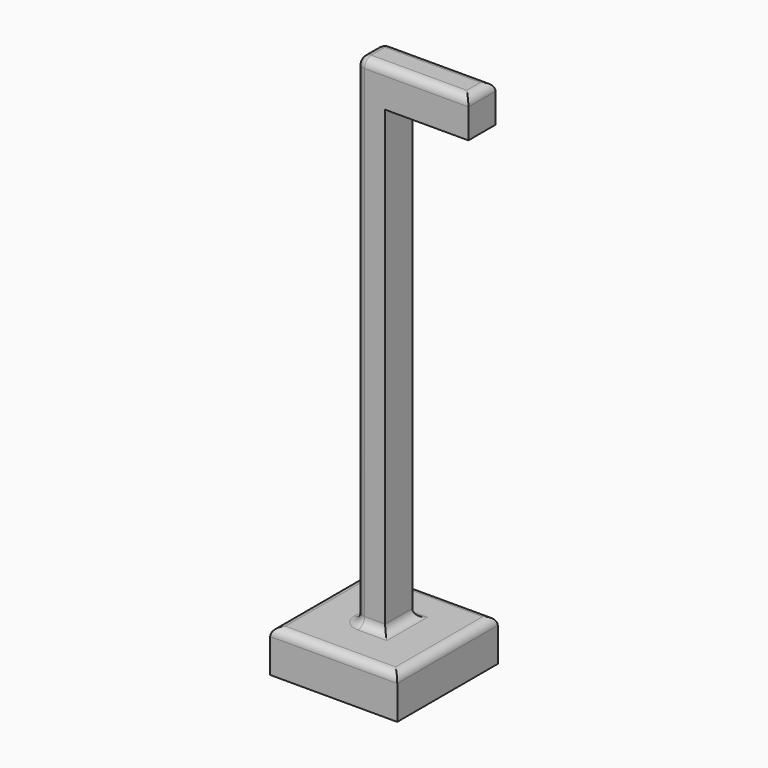
from build123d import *

# Parameters (mm, degrees)
F0_W        = 76.344192028
F0_H        = 75.5144134164
F1_DEPTH    = 25.4
F2_W        = 17.4319148064
F2_H        = 20.3372240067
F3_DEPTH    = 300
F4_W        = 20.3372240067
F4_H        = 22.7871290684
F5_DEPTH    = 50
F6_F1_R     = 5.08
F6_F2_R     = 5.08
F7_T        = 2.54
F7_T3_DEPTH = 10.16
F7_T5_DEPTH = 25.4172240067
F7_T7_DEPTH = 10.16
F8_R        = 5.08


# Not quite as in the source:
# - a shell that OpenCascade refuses in one call is made with other operations: the cavity is built on its own and cut out


with BuildPart() as f1:
    # F0 (on Top) → F1 (new body)
    with BuildSketch(Plane.XY):
        with Locations((38.172096014, 37.7572067082)):
            Rectangle(F0_W, F0_H)
    extrude(amount=F1_DEPTH)

    # F2 (on face) → F3 (join)
    with BuildSketch(Plane.XY.offset(25.4)):
        with Locations((37.6336574554, 38.5992005467)):
            Rectangle(F2_W, F2_H)
    extrude(amount=F3_DEPTH)

    # F4 (on face) → F5 (join)
    with BuildSketch(Plane.YZ.offset(46.3496148586)):
        with Locations((38.5992005467, 314.0064354658)):
            Rectangle(F4_W, F4_H)
    extrude(amount=F5_DEPTH)

    # F6: fillet of radius 5.08 on 7 edges, made by hand

    # F6_f1
    f6_f1_edges = [f1.edges().sort_by_distance(p)[0] for p in [
        (28.9177000523, 48.7678125501, 175.4),
        (28.9177000523, 28.4305885434, 175.4),
        (28.9177000523, 38.5992005467, 325.4),
        (62.6336574554, 48.7678125501, 325.4),
        (62.6336574554, 28.4305885434, 325.4),
        (96.3496148586, 38.5992005467, 325.4),
    ]]
    fillet(f6_f1_edges, radius=F6_F1_R)

    # F6_f2
    f6_f2_edges = [f1.edges().sort_by_distance(p)[0] for p in [
        (28.9177000523, 38.5992005467, 25.4),
        (30.4055976038, 47.2799149985, 25.4),
        (30.4055976038, 29.918486095, 25.4),
    ]]
    fillet(f6_f2_edges, radius=F6_F2_R)

    # F7: shell of thickness 2.54, made by hand


with BuildPart() as f7_core1:
    # F7_t2: copy of F1
    add(f1.part)

    # the walls: a layer under each face that stays
    f7_faces = [f7_core1.faces().sort_by_distance(p)[0] for p in [
        (12.7240320047, 12.5857355694, 25.4),
        (46.3496148586, 38.5992005467, 164.0064354658),
        (40.1736574554, 50.2557101016, 26.8878975516),
        (29.3534951554, 48.3320174469, 26.8878975516),
        (40.1736574554, 26.9426909918, 26.8878975516),
        (27.4298025007, 38.5992005467, 26.8878975516),
        (29.3534951554, 28.8663836466, 26.8878975516),
        (0, 37.7572067082, 12.7),
        (38.172096014, 75.5144134164, 12.7),
        (38.172096014, 0, 12.7),
        (76.344192028, 37.7572067082, 12.7),
        (44.3896858533, 48.7678125501, 272.0133333333),
        (44.3896858533, 28.4305885434, 272.0133333333),
        (30.4055976038, 47.2799149985, 175.4),
        (28.9177000523, 38.5992005467, 175.4),
        (30.4055976038, 29.918486095, 175.4),
        (38.172096014, 37.7572067082, 0),
        (65.1736574554, 47.2799149985, 323.9121024484),
        (96.3496148586, 38.5992005467, 311.4664354658),
        (65.1736574554, 29.918486095, 323.9121024484),
        (31.4577000523, 46.2278125501, 323.9121024484),
        (30.4055976038, 38.5992005467, 323.9121024484),
        (31.4577000523, 30.9705885434, 323.9121024484),
        (62.6336574554, 38.5992005467, 325.4),
        (94.8617173071, 38.5992005467, 323.9121024484),
    ]]
    thicken(f7_faces, amount=-F7_T, mode=Mode.SUBTRACT)

    # F7_s4 → F7_t3 (cut)
    with BuildSketch(Plane.XZ.offset(-56.3878125501)):
        Polygon((46.3750148586, 25.4254), (46.3496148586, 22.86), (43.8096148586, 22.86), (43.8096148586, 25.4), align=None)
    extrude(amount=F7_T3_DEPTH, mode=Mode.SUBTRACT)

    # F7_s6 → F7_t5 (cut)
    with BuildSketch(Plane.XZ.offset(-51.3078125501)):
        Polygon((46.3750148586, 25.4254), (46.3496148586, 22.86), (43.8096148586, 22.86), (43.8096148586, 25.4), align=None)
    extrude(amount=F7_T5_DEPTH, mode=Mode.SUBTRACT)

    # F7_s8 → F7_t7 (cut)
    with BuildSketch(Plane.XZ.offset(-30.9705885434)):
        Polygon((46.3750148586, 25.4254), (46.3496148586, 22.86), (43.8096148586, 22.86), (43.8096148586, 25.4), align=None)
    extrude(amount=F7_T7_DEPTH, mode=Mode.SUBTRACT)


with BuildPart() as f1_1:
    add(f1.part)

    # what is left inside the walls is the cavity
    f7_cavity = [f7_core1.part.solids().sort_by_distance(p)[0] for p in [
        (38.172096, 26.018138, 2.5654),
    ]]
    add(f7_cavity, mode=Mode.SUBTRACT)

    # F8
    f8_edges = [f1_1.edges().sort_by_distance(p)[0] for p in [
        (46.349615, 38.599201, 25.4),
        (40.173657, 23.350589, 25.4),
        (26.813495, 26.326384, 25.4),
        (23.8377, 38.599201, 25.4),
        (26.813495, 50.872017, 25.4),
        (40.173657, 53.847813, 25.4),
        (0, 37.757207, 25.4),
        (38.172096, 0, 25.4),
        (76.344192, 37.757207, 25.4),
        (38.172096, 75.514413, 25.4),
    ]]
    fillet(f8_edges, radius=F8_R)


solid = f1_1.part
